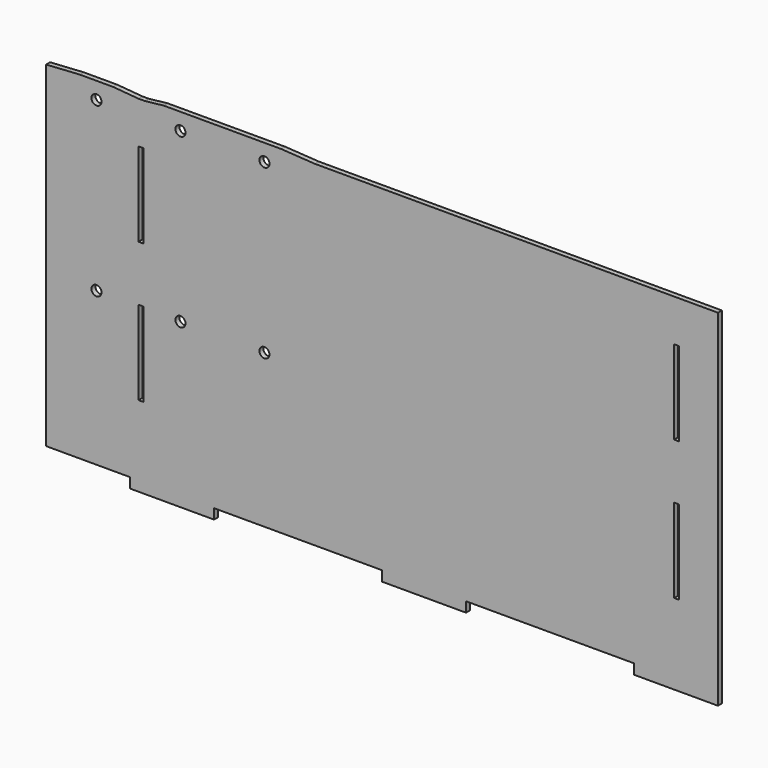
from build123d import *

# Parameters (mm, degrees)
F1_DEPTH  = 2.95
F2_W      = 2.95
F2_H      = 50
F3_DEPTH  = 2.95
F4_W      = 20
F4_H      = 2.95
F5_DEPTH  = 1.25
F7_D      = 6
F7_DEPTH  = 4
F7_TIP    = 1.8025818571
F8_W      = 30
F8_H      = 1.25
F9_DEPTH  = 2.95
F10_W     = 2.95
F10_H     = 50
F11_DEPTH = 2.95


# Not quite as in the source:
# - a feature names something its author has since deleted; it is built from what else it names


with BuildPart() as f1:
    # F0 (on Front) → F1 (new body)
    with BuildSketch(Plane.XZ):
        Polygon((50, -6), (50, 0), (150, 0), (150, -6), (200, -6), (200, 0), (300, 0), (300, -6), (350, -6), (350, 0), (350, 200), (0, 200), (-50, 200), (-50, 0), (0, 0), (0, -6), align=None)
    extrude(amount=F1_DEPTH)

    # F2 (on face) → F3 (cut)
    with BuildSketch(Plane.XZ.offset(2.95)):
        with Locations((325.4, 150)):
            Rectangle(F2_W, F2_H)
        with Locations((325.4, 67)):
            Rectangle(F2_W, F2_H)
    extrude(amount=-F3_DEPTH, mode=Mode.SUBTRACT)

    # F4 (on face) → F5 (join)
    with BuildSketch(Plane.XY.offset(200)):
        with Locations((80, -1.475)):
            Rectangle(F4_W, F4_H)
        with Locations((30, -1.475)):
            Rectangle(F4_W, F4_H)
        with Locations((-20, -1.475)):
            Rectangle(F4_W, F4_H)
    extrude(amount=F5_DEPTH)

    # F7
    with Locations(Plane(origin=(0, 0, 0), x_dir=(-1, 0, 0), z_dir=(0, 1, 0))):
        with Locations((-80, 91.25), (-80, 191.25), (-30, 91.25), (20, 91.25), (20, 191.25), (-30, 191.25)):
            Hole(F7_D / 2, depth=F7_DEPTH)
            with Locations((0, 0, -(F7_DEPTH + F7_TIP / 2))):  # 118° drill point
                Cone(0, F7_D / 2, F7_TIP, mode=Mode.SUBTRACT)

    # F8 (on face) → F9 (join)
    with BuildSketch(Plane(origin=(0, 0, 0), x_dir=(-1, 0, 0), z_dir=(0, 1, 0))):
        with Locations((-55, 200.625)):
            Rectangle(F8_W, F8_H)
        Polygon((30, 201.25), (30, 200), (50, 200), align=None)
        Polygon((-90, 200), (-90, 201.25), (-110, 200), align=None)
        Polygon((10, 201.25), (-5, 200), (10, 200), align=None)
        Polygon((-8.75, 200), (-20, 201.25), (-20, 200), align=None)
    extrude(amount=-F9_DEPTH)

    # F10 (on face) → F11 (cut)
    with BuildSketch(Plane(origin=(0, 0, 0), x_dir=(-1, 0, 0), z_dir=(0, 1, 0))):
        with Locations((-6.475, 150)):
            Rectangle(F10_W, F10_H)
        with Locations((-6.475, 67)):
            Rectangle(F10_W, F10_H)
    extrude(amount=-F11_DEPTH, mode=Mode.SUBTRACT)


solid = f1.part
